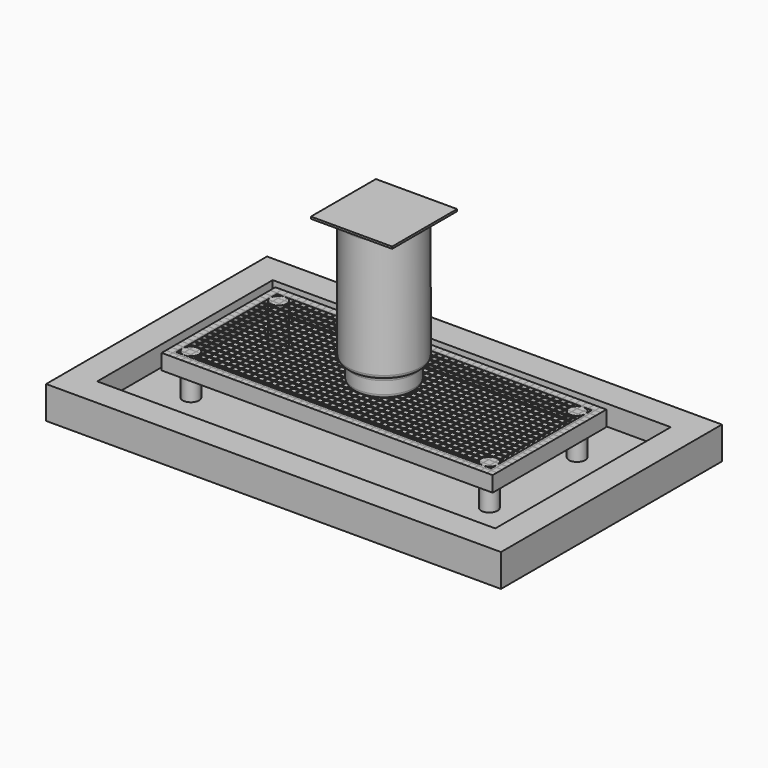
from build123d import *

# Parameters (mm, degrees)
F1_W      = 560
F1_H      = 340
F2_DEPTH  = 40
F3_T      = -35
F4_W      = 490
F4_H      = 270
F5_DEPTH  = 20
F6_R      = 10
F7_DEPTH  = 50
F8_W      = 407.5
F8_H      = 175
F9_DEPTH  = 19.05
F10_W     = 407.5
F10_H     = 0.5
F11_DEPTH = 1
F12_W     = 0.5
F12_H     = 175
F13_DEPTH = 1
F14_R     = 37.5
F15_DEPTH = 25
F16_R     = 45
F17_DEPTH = 155
F18_R     = 5
F19_R     = 5
F20_W     = 100
F20_H     = 100
F21_DEPTH = 2.5


with BuildPart() as f2:
    # F1 (on offset) → F2 (new body)
    with BuildSketch(Plane.XY.offset(-167.5)):
        Rectangle(F1_W, F1_H)
    extrude(amount=F2_DEPTH)

    # F3
    f3_openings = [f2.faces().sort_by_distance(p)[0] for p in [
        (0, 0, -127.5),
    ]]
    offset(amount=F3_T, openings=f3_openings)

    # F4 (on face) → F5 (cut)
    with BuildSketch(Plane.XY.offset(-132.5)):
        Rectangle(F4_W, F4_H)
    extrude(amount=-F5_DEPTH, mode=Mode.SUBTRACT)

    # F6 (on face) → F7 (join)
    with BuildSketch(Plane.XY.offset(-152.5)):
        with Locations((-183.75, 67.5)):
            Circle(F6_R)
        with Locations((183.75, 67.5)):
            Circle(F6_R)
        with Locations((-183.75, -67.5)):
            Circle(F6_R)
        with Locations((183.75, -67.5)):
            Circle(F6_R)
    extrude(amount=F7_DEPTH)

    # F8 (on face) → F9 (join)
    with BuildSketch(Plane.XY.offset(-102.5)):
        Rectangle(F8_W, F8_H)
        Polygon((-193.75, 77.5), (-183.75, 77.5), (193.75, 77.5), (193.75, -77.5), (-193.75, -77.5), (-193.75, 67.5), align=None, mode=Mode.SUBTRACT)
    extrude(amount=-F9_DEPTH)


with BuildPart() as f11:
    # F10 (on face) → F11 (new body)
    with BuildSketch(Plane.XY.offset(-102.5)):
        with Locations((0, 87.25)):
            Rectangle(F10_W, F10_H)
    extrude(amount=-F11_DEPTH)


with BuildPart() as f11b:
    # F10 (on face) → F11, piece 2 (new body)
    with BuildSketch(Plane.XY.offset(-102.5)):
        with Locations((0, 79.25)):
            Rectangle(F10_W, F10_H)
    extrude(amount=-F11_DEPTH)


with BuildPart() as f11c:
    # F10 (on face) → F11, piece 3 (new body)
    with BuildSketch(Plane.XY.offset(-102.5)):
        with Locations((0, 71.25)):
            Rectangle(F10_W, F10_H)
    extrude(amount=-F11_DEPTH)


with BuildPart() as f11d:
    # F10 (on face) → F11, piece 4 (new body)
    with BuildSketch(Plane.XY.offset(-102.5)):
        with Locations((0, 63.25)):
            Rectangle(F10_W, F10_H)
    extrude(amount=-F11_DEPTH)


with BuildPart() as f11e:
    # F10 (on face) → F11, piece 5 (new body)
    with BuildSketch(Plane.XY.offset(-102.5)):
        with Locations((0, 55.25)):
            Rectangle(F10_W, F10_H)
    extrude(amount=-F11_DEPTH)


with BuildPart() as f11f:
    # F10 (on face) → F11, piece 6 (new body)
    with BuildSketch(Plane.XY.offset(-102.5)):
        with Locations((0, 47.25)):
            Rectangle(F10_W, F10_H)
    extrude(amount=-F11_DEPTH)


with BuildPart() as f11g:
    # F10 (on face) → F11, piece 7 (new body)
    with BuildSketch(Plane.XY.offset(-102.5)):
        with Locations((0, 39.25)):
            Rectangle(F10_W, F10_H)
    extrude(amount=-F11_DEPTH)


with BuildPart() as f11h:
    # F10 (on face) → F11, piece 8 (new body)
    with BuildSketch(Plane.XY.offset(-102.5)):
        with Locations((0, 31.25)):
            Rectangle(F10_W, F10_H)
    extrude(amount=-F11_DEPTH)


with BuildPart() as f11i:
    # F10 (on face) → F11, piece 9 (new body)
    with BuildSketch(Plane.XY.offset(-102.5)):
        with Locations((0, 23.25)):
            Rectangle(F10_W, F10_H)
    extrude(amount=-F11_DEPTH)


with BuildPart() as f11j:
    # F10 (on face) → F11, piece 10 (new body)
    with BuildSketch(Plane.XY.offset(-102.5)):
        with Locations((0, 15.25)):
            Rectangle(F10_W, F10_H)
    extrude(amount=-F11_DEPTH)


with BuildPart() as f11k:
    # F10 (on face) → F11, piece 11 (new body)
    with BuildSketch(Plane.XY.offset(-102.5)):
        with Locations((0, 7.25)):
            Rectangle(F10_W, F10_H)
    extrude(amount=-F11_DEPTH)


with BuildPart() as f11l:
    # F10 (on face) → F11, piece 12 (new body)
    with BuildSketch(Plane.XY.offset(-102.5)):
        with Locations((0, -0.75)):
            Rectangle(F10_W, F10_H)
    extrude(amount=-F11_DEPTH)


with BuildPart() as f11m:
    # F10 (on face) → F11, piece 13 (new body)
    with BuildSketch(Plane.XY.offset(-102.5)):
        with Locations((0, -8.75)):
            Rectangle(F10_W, F10_H)
    extrude(amount=-F11_DEPTH)


with BuildPart() as f11n:
    # F10 (on face) → F11, piece 14 (new body)
    with BuildSketch(Plane.XY.offset(-102.5)):
        with Locations((0, -16.75)):
            Rectangle(F10_W, F10_H)
    extrude(amount=-F11_DEPTH)


with BuildPart() as f11o:
    # F10 (on face) → F11, piece 15 (new body)
    with BuildSketch(Plane.XY.offset(-102.5)):
        with Locations((0, -24.75)):
            Rectangle(F10_W, F10_H)
    extrude(amount=-F11_DEPTH)


with BuildPart() as f11p:
    # F10 (on face) → F11, piece 16 (new body)
    with BuildSketch(Plane.XY.offset(-102.5)):
        with Locations((0, -32.75)):
            Rectangle(F10_W, F10_H)
    extrude(amount=-F11_DEPTH)


with BuildPart() as f11q:
    # F10 (on face) → F11, piece 17 (new body)
    with BuildSketch(Plane.XY.offset(-102.5)):
        with Locations((0, -40.75)):
            Rectangle(F10_W, F10_H)
    extrude(amount=-F11_DEPTH)


with BuildPart() as f11r:
    # F10 (on face) → F11, piece 18 (new body)
    with BuildSketch(Plane.XY.offset(-102.5)):
        with Locations((0, -48.75)):
            Rectangle(F10_W, F10_H)
    extrude(amount=-F11_DEPTH)


with BuildPart() as f11s:
    # F10 (on face) → F11, piece 19 (new body)
    with BuildSketch(Plane.XY.offset(-102.5)):
        with Locations((0, -56.75)):
            Rectangle(F10_W, F10_H)
    extrude(amount=-F11_DEPTH)


with BuildPart() as f11t:
    # F10 (on face) → F11, piece 20 (new body)
    with BuildSketch(Plane.XY.offset(-102.5)):
        with Locations((0, -64.75)):
            Rectangle(F10_W, F10_H)
    extrude(amount=-F11_DEPTH)


with BuildPart() as f11u:
    # F10 (on face) → F11, piece 21 (new body)
    with BuildSketch(Plane.XY.offset(-102.5)):
        with Locations((0, -72.75)):
            Rectangle(F10_W, F10_H)
    extrude(amount=-F11_DEPTH)


with BuildPart() as f11v:
    # F10 (on face) → F11, piece 22 (new body)
    with BuildSketch(Plane.XY.offset(-102.5)):
        with Locations((0, -80.75)):
            Rectangle(F10_W, F10_H)
    extrude(amount=-F11_DEPTH)


with BuildPart() as f13:
    # F12 (on face) → F13 (new body)
    with BuildSketch(Plane.XY.offset(-102.5)):
        with Locations((-203.5, 0)):
            Rectangle(F12_W, F12_H)
    extrude(amount=-F13_DEPTH)


with BuildPart() as f13b:
    # F12 (on face) → F13, piece 2 (new body)
    with BuildSketch(Plane.XY.offset(-102.5)):
        with Locations((-195.5, 0)):
            Rectangle(F12_W, F12_H)
    extrude(amount=-F13_DEPTH)


with BuildPart() as f13c:
    # F12 (on face) → F13, piece 3 (new body)
    with BuildSketch(Plane.XY.offset(-102.5)):
        with Locations((-187.5, 0)):
            Rectangle(F12_W, F12_H)
    extrude(amount=-F13_DEPTH)


with BuildPart() as f13d:
    # F12 (on face) → F13, piece 4 (new body)
    with BuildSketch(Plane.XY.offset(-102.5)):
        with Locations((-179.5, 0)):
            Rectangle(F12_W, F12_H)
    extrude(amount=-F13_DEPTH)


with BuildPart() as f13e:
    # F12 (on face) → F13, piece 5 (new body)
    with BuildSketch(Plane.XY.offset(-102.5)):
        with Locations((-171.5, 0)):
            Rectangle(F12_W, F12_H)
    extrude(amount=-F13_DEPTH)


with BuildPart() as f13f:
    # F12 (on face) → F13, piece 6 (new body)
    with BuildSketch(Plane.XY.offset(-102.5)):
        with Locations((-163.5, 0)):
            Rectangle(F12_W, F12_H)
    extrude(amount=-F13_DEPTH)


with BuildPart() as f13g:
    # F12 (on face) → F13, piece 7 (new body)
    with BuildSketch(Plane.XY.offset(-102.5)):
        with Locations((-155.5, 0)):
            Rectangle(F12_W, F12_H)
    extrude(amount=-F13_DEPTH)


with BuildPart() as f13h:
    # F12 (on face) → F13, piece 8 (new body)
    with BuildSketch(Plane.XY.offset(-102.5)):
        with Locations((-147.5, 0)):
            Rectangle(F12_W, F12_H)
    extrude(amount=-F13_DEPTH)


with BuildPart() as f13i:
    # F12 (on face) → F13, piece 9 (new body)
    with BuildSketch(Plane.XY.offset(-102.5)):
        with Locations((-139.5, 0)):
            Rectangle(F12_W, F12_H)
    extrude(amount=-F13_DEPTH)


with BuildPart() as f13j:
    # F12 (on face) → F13, piece 10 (new body)
    with BuildSketch(Plane.XY.offset(-102.5)):
        with Locations((-131.5, 0)):
            Rectangle(F12_W, F12_H)
    extrude(amount=-F13_DEPTH)


with BuildPart() as f13k:
    # F12 (on face) → F13, piece 11 (new body)
    with BuildSketch(Plane.XY.offset(-102.5)):
        with Locations((-123.5, 0)):
            Rectangle(F12_W, F12_H)
    extrude(amount=-F13_DEPTH)


with BuildPart() as f13l:
    # F12 (on face) → F13, piece 12 (new body)
    with BuildSketch(Plane.XY.offset(-102.5)):
        with Locations((-115.5, 0)):
            Rectangle(F12_W, F12_H)
    extrude(amount=-F13_DEPTH)


with BuildPart() as f13m:
    # F12 (on face) → F13, piece 13 (new body)
    with BuildSketch(Plane.XY.offset(-102.5)):
        with Locations((-107.5, 0)):
            Rectangle(F12_W, F12_H)
    extrude(amount=-F13_DEPTH)


with BuildPart() as f13n:
    # F12 (on face) → F13, piece 14 (new body)
    with BuildSketch(Plane.XY.offset(-102.5)):
        with Locations((-99.5, 0)):
            Rectangle(F12_W, F12_H)
    extrude(amount=-F13_DEPTH)


with BuildPart() as f13o:
    # F12 (on face) → F13, piece 15 (new body)
    with BuildSketch(Plane.XY.offset(-102.5)):
        with Locations((-91.5, 0)):
            Rectangle(F12_W, F12_H)
    extrude(amount=-F13_DEPTH)


with BuildPart() as f13p:
    # F12 (on face) → F13, piece 16 (new body)
    with BuildSketch(Plane.XY.offset(-102.5)):
        with Locations((-83.5, 0)):
            Rectangle(F12_W, F12_H)
    extrude(amount=-F13_DEPTH)


with BuildPart() as f13q:
    # F12 (on face) → F13, piece 17 (new body)
    with BuildSketch(Plane.XY.offset(-102.5)):
        with Locations((-75.5, 0)):
            Rectangle(F12_W, F12_H)
    extrude(amount=-F13_DEPTH)


with BuildPart() as f13r:
    # F12 (on face) → F13, piece 18 (new body)
    with BuildSketch(Plane.XY.offset(-102.5)):
        with Locations((-67.5, 0)):
            Rectangle(F12_W, F12_H)
    extrude(amount=-F13_DEPTH)


with BuildPart() as f13s:
    # F12 (on face) → F13, piece 19 (new body)
    with BuildSketch(Plane.XY.offset(-102.5)):
        with Locations((-59.5, 0)):
            Rectangle(F12_W, F12_H)
    extrude(amount=-F13_DEPTH)


with BuildPart() as f13t:
    # F12 (on face) → F13, piece 20 (new body)
    with BuildSketch(Plane.XY.offset(-102.5)):
        with Locations((-51.5, 0)):
            Rectangle(F12_W, F12_H)
    extrude(amount=-F13_DEPTH)


with BuildPart() as f13u:
    # F12 (on face) → F13, piece 21 (new body)
    with BuildSketch(Plane.XY.offset(-102.5)):
        with Locations((-43.5, 0)):
            Rectangle(F12_W, F12_H)
    extrude(amount=-F13_DEPTH)


with BuildPart() as f13v:
    # F12 (on face) → F13, piece 22 (new body)
    with BuildSketch(Plane.XY.offset(-102.5)):
        with Locations((-35.5, 0)):
            Rectangle(F12_W, F12_H)
    extrude(amount=-F13_DEPTH)


with BuildPart() as f13w:
    # F12 (on face) → F13, piece 23 (new body)
    with BuildSketch(Plane.XY.offset(-102.5)):
        with Locations((-27.5, 0)):
            Rectangle(F12_W, F12_H)
    extrude(amount=-F13_DEPTH)


with BuildPart() as f13x:
    # F12 (on face) → F13, piece 24 (new body)
    with BuildSketch(Plane.XY.offset(-102.5)):
        with Locations((-19.5, 0)):
            Rectangle(F12_W, F12_H)
    extrude(amount=-F13_DEPTH)


with BuildPart() as f13y:
    # F12 (on face) → F13, piece 25 (new body)
    with BuildSketch(Plane.XY.offset(-102.5)):
        with Locations((-11.5, 0)):
            Rectangle(F12_W, F12_H)
    extrude(amount=-F13_DEPTH)


with BuildPart() as f13z:
    # F12 (on face) → F13, piece 26 (new body)
    with BuildSketch(Plane.XY.offset(-102.5)):
        with Locations((-3.5, 0)):
            Rectangle(F12_W, F12_H)
    extrude(amount=-F13_DEPTH)


with BuildPart() as f13ba:
    # F12 (on face) → F13, piece 27 (new body)
    with BuildSketch(Plane.XY.offset(-102.5)):
        with Locations((4.5, 0)):
            Rectangle(F12_W, F12_H)
    extrude(amount=-F13_DEPTH)


with BuildPart() as f13bb:
    # F12 (on face) → F13, piece 28 (new body)
    with BuildSketch(Plane.XY.offset(-102.5)):
        with Locations((12.5, 0)):
            Rectangle(F12_W, F12_H)
    extrude(amount=-F13_DEPTH)


with BuildPart() as f13bc:
    # F12 (on face) → F13, piece 29 (new body)
    with BuildSketch(Plane.XY.offset(-102.5)):
        with Locations((20.5, 0)):
            Rectangle(F12_W, F12_H)
    extrude(amount=-F13_DEPTH)


with BuildPart() as f13bd:
    # F12 (on face) → F13, piece 30 (new body)
    with BuildSketch(Plane.XY.offset(-102.5)):
        with Locations((28.5, 0)):
            Rectangle(F12_W, F12_H)
    extrude(amount=-F13_DEPTH)


with BuildPart() as f13be:
    # F12 (on face) → F13, piece 31 (new body)
    with BuildSketch(Plane.XY.offset(-102.5)):
        with Locations((36.5, 0)):
            Rectangle(F12_W, F12_H)
    extrude(amount=-F13_DEPTH)


with BuildPart() as f13bf:
    # F12 (on face) → F13, piece 32 (new body)
    with BuildSketch(Plane.XY.offset(-102.5)):
        with Locations((44.5, 0)):
            Rectangle(F12_W, F12_H)
    extrude(amount=-F13_DEPTH)


with BuildPart() as f13bg:
    # F12 (on face) → F13, piece 33 (new body)
    with BuildSketch(Plane.XY.offset(-102.5)):
        with Locations((52.5, 0)):
            Rectangle(F12_W, F12_H)
    extrude(amount=-F13_DEPTH)


with BuildPart() as f13bh:
    # F12 (on face) → F13, piece 34 (new body)
    with BuildSketch(Plane.XY.offset(-102.5)):
        with Locations((60.5, 0)):
            Rectangle(F12_W, F12_H)
    extrude(amount=-F13_DEPTH)


with BuildPart() as f13bi:
    # F12 (on face) → F13, piece 35 (new body)
    with BuildSketch(Plane.XY.offset(-102.5)):
        with Locations((68.5, 0)):
            Rectangle(F12_W, F12_H)
    extrude(amount=-F13_DEPTH)


with BuildPart() as f13bj:
    # F12 (on face) → F13, piece 36 (new body)
    with BuildSketch(Plane.XY.offset(-102.5)):
        with Locations((76.5, 0)):
            Rectangle(F12_W, F12_H)
    extrude(amount=-F13_DEPTH)


with BuildPart() as f13bk:
    # F12 (on face) → F13, piece 37 (new body)
    with BuildSketch(Plane.XY.offset(-102.5)):
        with Locations((84.5, 0)):
            Rectangle(F12_W, F12_H)
    extrude(amount=-F13_DEPTH)


with BuildPart() as f13bl:
    # F12 (on face) → F13, piece 38 (new body)
    with BuildSketch(Plane.XY.offset(-102.5)):
        with Locations((92.5, 0)):
            Rectangle(F12_W, F12_H)
    extrude(amount=-F13_DEPTH)


with BuildPart() as f13bm:
    # F12 (on face) → F13, piece 39 (new body)
    with BuildSketch(Plane.XY.offset(-102.5)):
        with Locations((100.5, 0)):
            Rectangle(F12_W, F12_H)
    extrude(amount=-F13_DEPTH)


with BuildPart() as f13bn:
    # F12 (on face) → F13, piece 40 (new body)
    with BuildSketch(Plane.XY.offset(-102.5)):
        with Locations((108.5, 0)):
            Rectangle(F12_W, F12_H)
    extrude(amount=-F13_DEPTH)


with BuildPart() as f13bo:
    # F12 (on face) → F13, piece 41 (new body)
    with BuildSketch(Plane.XY.offset(-102.5)):
        with Locations((116.5, 0)):
            Rectangle(F12_W, F12_H)
    extrude(amount=-F13_DEPTH)


with BuildPart() as f13bp:
    # F12 (on face) → F13, piece 42 (new body)
    with BuildSketch(Plane.XY.offset(-102.5)):
        with Locations((124.5, 0)):
            Rectangle(F12_W, F12_H)
    extrude(amount=-F13_DEPTH)


with BuildPart() as f13bq:
    # F12 (on face) → F13, piece 43 (new body)
    with BuildSketch(Plane.XY.offset(-102.5)):
        with Locations((132.5, 0)):
            Rectangle(F12_W, F12_H)
    extrude(amount=-F13_DEPTH)


with BuildPart() as f13br:
    # F12 (on face) → F13, piece 44 (new body)
    with BuildSketch(Plane.XY.offset(-102.5)):
        with Locations((140.5, 0)):
            Rectangle(F12_W, F12_H)
    extrude(amount=-F13_DEPTH)


with BuildPart() as f13bs:
    # F12 (on face) → F13, piece 45 (new body)
    with BuildSketch(Plane.XY.offset(-102.5)):
        with Locations((148.5, 0)):
            Rectangle(F12_W, F12_H)
    extrude(amount=-F13_DEPTH)


with BuildPart() as f13bt:
    # F12 (on face) → F13, piece 46 (new body)
    with BuildSketch(Plane.XY.offset(-102.5)):
        with Locations((156.5, 0)):
            Rectangle(F12_W, F12_H)
    extrude(amount=-F13_DEPTH)


with BuildPart() as f13bu:
    # F12 (on face) → F13, piece 47 (new body)
    with BuildSketch(Plane.XY.offset(-102.5)):
        with Locations((164.5, 0)):
            Rectangle(F12_W, F12_H)
    extrude(amount=-F13_DEPTH)


with BuildPart() as f13bv:
    # F12 (on face) → F13, piece 48 (new body)
    with BuildSketch(Plane.XY.offset(-102.5)):
        with Locations((172.5, 0)):
            Rectangle(F12_W, F12_H)
    extrude(amount=-F13_DEPTH)


with BuildPart() as f13bw:
    # F12 (on face) → F13, piece 49 (new body)
    with BuildSketch(Plane.XY.offset(-102.5)):
        with Locations((180.5, 0)):
            Rectangle(F12_W, F12_H)
    extrude(amount=-F13_DEPTH)


with BuildPart() as f13bx:
    # F12 (on face) → F13, piece 50 (new body)
    with BuildSketch(Plane.XY.offset(-102.5)):
        with Locations((188.5, 0)):
            Rectangle(F12_W, F12_H)
    extrude(amount=-F13_DEPTH)


with BuildPart() as f13by:
    # F12 (on face) → F13, piece 51 (new body)
    with BuildSketch(Plane.XY.offset(-102.5)):
        with Locations((196.5, 0)):
            Rectangle(F12_W, F12_H)
    extrude(amount=-F13_DEPTH)


with BuildPart() as f15:
    # F14 (on face) → F15 (new body)
    with BuildSketch(Plane.XY.offset(-102.5)):
        Circle(F14_R)
    extrude(amount=F15_DEPTH)

    # F16 (on face) → F17 (join)
    with BuildSketch(Plane.XY.offset(-77.5)):
        Circle(F16_R)
    extrude(amount=F17_DEPTH)

    # F18
    f18_edges = [f15.edges().sort_by_distance(p)[0] for p in [
        (-37.5, 0, -102.5),
        (-45, 0, 77.5),
        (-37.5, 0, -77.5),
    ]]
    fillet(f18_edges, radius=F18_R)

    # F19
    f19_edges = [f15.edges().sort_by_distance(p)[0] for p in [
        (-45, 0, -77.5),
    ]]
    fillet(f19_edges, radius=F19_R)

    # F20 (on face) → F21 (join)
    with BuildSketch(Plane.XY.offset(77.5)):
        Rectangle(F20_W, F20_H)
    extrude(amount=F21_DEPTH)


solid = Compound([f2.part, f11.part, f11b.part, f11c.part, f11d.part, f11e.part, f11f.part, f11g.part, f11h.part, f11i.part, f11j.part, f11k.part, f11l.part, f11m.part, f11n.part, f11o.part, f11p.part, f11q.part, f11r.part, f11s.part, f11t.part, f11u.part, f11v.part, f13.part, f13b.part, f13c.part, f13d.part, f13e.part, f13f.part, f13g.part, f13h.part, f13i.part, f13j.part, f13k.part, f13l.part, f13m.part, f13n.part, f13o.part, f13p.part, f13q.part, f13r.part, f13s.part, f13t.part, f13u.part, f13v.part, f13w.part, f13x.part, f13y.part, f13z.part, f13ba.part, f13bb.part, f13bc.part, f13bd.part, f13be.part, f13bf.part, f13bg.part, f13bh.part, f13bi.part, f13bj.part, f13bk.part, f13bl.part, f13bm.part, f13bn.part, f13bo.part, f13bp.part, f13bq.part, f13br.part, f13bs.part, f13bt.part, f13bu.part, f13bv.part, f13bw.part, f13bx.part, f13by.part, f15.part])
